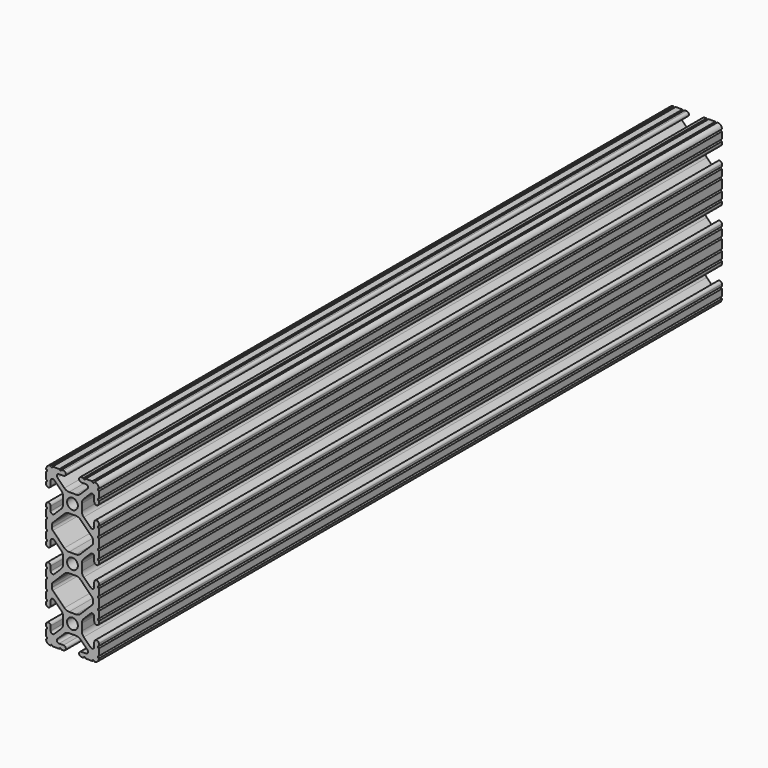
from build123d import *

# Parameters (mm, degrees)
F1_DEPTH = 375


# Not quite as in the source:
# - ends of sketch curves that miss each other by under 0.0002 mm in the source are joined


with BuildPart() as f1:
    # F0 (on Front) → F1 (new body)
    with BuildSketch(Plane.XZ):
        with BuildLine():
            ThreePointArc((-9.5504, 38.1), (-10.0584, 37.592), (-10.5664, 38.1))
            ThreePointArc((-10.5664, 38.1), (-12.0826749161, 37.4826749161), (-12.699997541, 35.9664000298))
            ThreePointArc((-12.699997541, 35.9664000298), (-12.192, 35.4584), (-12.7, 34.9504))
            Line((-12.7, 34.9504), (-12.7, 31.7246))
            ThreePointArc((-12.7, 31.7246), (-12.192, 31.2166), (-12.7, 30.7086))
            Line((-12.7, 30.7086), (-12.7, 29.7023028))
            ThreePointArc((-12.7, 29.7023028), (-11.5951, 28.5974028), (-10.4902, 29.7023028))
            Line((-10.4902, 29.7023028), (-10.4902, 31.8747902))
            ThreePointArc((-10.4902, 31.8747902), (-9.8630063673, 32.813451805), (-8.7557795103, 32.5932106897))
            Line((-8.7557795103, 32.5932106897), (-5.4384448, 29.2758622))
            ThreePointArc((-5.4384448, 29.2758622), (-4.7501824843, 28.2458268978), (-4.5085, 27.030807))
            Line((-4.5085, 27.030807), (-4.5085, 23.769193))
            ThreePointArc((-4.5085, 23.769193), (-4.7501824843, 22.5541731022), (-5.4384359697, 21.5241289697))
            Line((-5.4384359697, 21.5241289697), (-8.7557864, 18.2067962))
            ThreePointArc((-8.7557864, 18.2067962), (-9.8630063673, 17.986548195), (-10.4902, 18.9252098))
            Line((-10.4902, 18.9252098), (-10.4902, 21.0976972))
            ThreePointArc((-10.4902, 21.0976972), (-11.5951, 22.2025972), (-12.7, 21.0976972))
            Line((-12.7, 21.0976972), (-12.7, 20.0914))
            ThreePointArc((-12.7, 20.0914), (-12.192, 19.5834), (-12.7, 19.0754))
            Line((-12.7, 19.0754), (-12.7, 15.8496))
            ThreePointArc((-12.7, 15.8496), (-12.192, 15.3416), (-12.7, 14.8336))
            Line((-12.7, 14.8336), (-12.7, 10.5664))
            ThreePointArc((-12.7, 10.5664), (-12.192, 10.0584), (-12.7, 9.5504))
            Line((-12.7, 9.5504), (-12.7, 6.3246))
            ThreePointArc((-12.7, 6.3246), (-12.192, 5.8166), (-12.7, 5.3086))
            Line((-12.7, 5.3086), (-12.7, 4.3023028))
            ThreePointArc((-12.7, 4.3023028), (-11.5951, 3.1974028), (-10.4902, 4.3023028))
            Line((-10.4902, 4.3023028), (-10.4902, 6.4747902))
            ThreePointArc((-10.4902, 6.4747902), (-9.8630063673, 7.413451805), (-8.7557795103, 7.1932106897))
            Line((-8.7557795103, 7.1932106897), (-5.4384448, 3.8758622))
            ThreePointArc((-5.4384448, 3.8758622), (-4.7501824843, 2.8458268978), (-4.5085, 1.630807))
            Line((-4.5085, 1.630807), (-4.5085, -1.630807))
            ThreePointArc((-4.5085, -1.630807), (-4.7501824843, -2.8458268978), (-5.4384359697, -3.8758710303))
            Line((-5.4384359697, -3.8758710303), (-8.7557864, -7.1932038))
            ThreePointArc((-8.7557864, -7.1932038), (-9.8630063673, -7.413451805), (-10.4902, -6.4747902))
            Line((-10.4902, -6.4747902), (-10.4902, -4.3023028))
            ThreePointArc((-10.4902, -4.3023028), (-11.5951, -3.1974028), (-12.7, -4.3023028))
            Line((-12.7, -4.3023028), (-12.7, -5.3086))
            ThreePointArc((-12.7, -5.3086), (-12.192, -5.8166), (-12.7, -6.3246))
            Line((-12.7, -6.3246), (-12.7, -9.5504))
            ThreePointArc((-12.7, -9.5504), (-12.192, -10.0584), (-12.7, -10.5664))
            Line((-12.7, -10.5664), (-12.7, -14.8336))
            ThreePointArc((-12.7, -14.8336), (-12.192, -15.3416), (-12.7, -15.8496))
            Line((-12.7, -15.8496), (-12.7, -19.0754))
            ThreePointArc((-12.7, -19.0754), (-12.192, -19.5834), (-12.7, -20.0914))
            Line((-12.7, -20.0914), (-12.7, -21.0976972))
            ThreePointArc((-12.7, -21.0976972), (-11.5951, -22.2025972), (-10.4902, -21.0976972))
            Line((-10.4902, -21.0976972), (-10.4902, -18.9252098))
            ThreePointArc((-10.4902, -18.9252098), (-9.8630063673, -17.986548195), (-8.7557795103, -18.2067893103))
            Line((-8.7557795103, -18.2067893103), (-5.4384448, -21.5241378))
            ThreePointArc((-5.4384448, -21.5241378), (-4.7501824843, -22.5541731022), (-4.5085, -23.769193))
            Line((-4.5085, -23.769193), (-4.5085, -27.030807))
            ThreePointArc((-4.5085, -27.030807), (-4.7501824843, -28.2458268978), (-5.4384359697, -29.2758710303))
            Line((-5.4384359697, -29.2758710303), (-8.7557864, -32.5932038))
            ThreePointArc((-8.7557864, -32.5932038), (-9.8630063673, -32.813451805), (-10.4902, -31.8747902))
            Line((-10.4902, -31.8747902), (-10.4902, -29.7023028))
            ThreePointArc((-10.4902, -29.7023028), (-11.5951, -28.5974028), (-12.7, -29.7023028))
            Line((-12.7, -29.7023028), (-12.7, -30.7086))
            ThreePointArc((-12.7, -30.7086), (-12.192, -31.2166), (-12.7, -31.7246))
            Line((-12.7, -31.7246), (-12.7, -34.9504))
            ThreePointArc((-12.7, -34.9504), (-12.192, -35.4584), (-12.7, -35.9664))
            ThreePointArc((-12.7, -35.9664), (-12.0826749161, -37.4826749161), (-10.5664000298, -38.099997541))
            ThreePointArc((-10.5664000298, -38.099997541), (-10.0584, -37.592), (-9.5504, -38.1))
            Line((-9.5504, -38.1), (-6.3246, -38.1))
            ThreePointArc((-6.3246, -38.1), (-5.8166, -37.592), (-5.3086, -38.1))
            Line((-5.3086, -38.1), (-4.3023028, -38.1))
            ThreePointArc((-4.3023028, -38.1), (-3.1974028, -36.9951), (-4.3023028, -35.8902))
            Line((-4.3023028, -35.8902), (-6.4747902, -35.8902))
            ThreePointArc((-6.4747902, -35.8902), (-7.413451805, -35.2630063673), (-7.1932106897, -34.1557795103))
            Line((-7.1932106897, -34.1557795103), (-3.8758622, -30.8384448))
            ThreePointArc((-3.8758622, -30.8384448), (-2.8458268978, -30.1501824843), (-1.630807, -29.9085))
            Line((-1.630807, -29.9085), (1.630807, -29.9085))
            ThreePointArc((1.630807, -29.9085), (2.8458268978, -30.1501824843), (3.8758710303, -30.8384359697))
            Line((3.8758710303, -30.8384359697), (7.1932038, -34.1557864))
            ThreePointArc((7.1932038, -34.1557864), (7.413451805, -35.2630063673), (6.4747902, -35.8902))
            Line((6.4747902, -35.8902), (4.3023028, -35.8902))
            ThreePointArc((4.3023028, -35.8902), (3.1974028, -36.9951), (4.3023028, -38.1))
            Line((4.3023028, -38.1), (5.3086, -38.1))
            ThreePointArc((5.3086, -38.1), (5.8166, -37.592), (6.3246, -38.1))
            Line((6.3246, -38.1), (9.5504, -38.1))
            ThreePointArc((9.5504, -38.1), (10.0584, -37.592), (10.5664, -38.1))
            ThreePointArc((10.5664, -38.1), (12.0826749161, -37.4826749161), (12.699997541, -35.9664000298))
            ThreePointArc((12.699997541, -35.9664000298), (12.192, -35.4584), (12.7, -34.9504))
            Line((12.7, -34.9504), (12.7, -31.7246))
            ThreePointArc((12.7, -31.7246), (12.192, -31.2166), (12.7, -30.7086))
            Line((12.7, -30.7086), (12.7, -29.7023028))
            ThreePointArc((12.7, -29.7023028), (11.5951, -28.5974028), (10.4902, -29.7023028))
            Line((10.4902, -29.7023028), (10.4902, -31.8747902))
            ThreePointArc((10.4902, -31.8747902), (9.8630063673, -32.813451805), (8.7557795103, -32.5932106897))
            Line((8.7557795103, -32.5932106897), (5.4384448, -29.2758622))
            ThreePointArc((5.4384448, -29.2758622), (4.7501824843, -28.2458268978), (4.5085, -27.030807))
            Line((4.5085, -27.030807), (4.5085, -23.769193))
            ThreePointArc((4.5085, -23.769193), (4.7501824843, -22.5541731022), (5.4384359697, -21.5241289697))
            Line((5.4384359697, -21.5241289697), (8.7557864, -18.2067962))
            ThreePointArc((8.7557864, -18.2067962), (9.8630063673, -17.986548195), (10.4902, -18.9252098))
            Line((10.4902, -18.9252098), (10.4902, -21.0976972))
            ThreePointArc((10.4902, -21.0976972), (11.5951, -22.2025972), (12.7, -21.0976972))
            Line((12.7, -21.0976972), (12.7, -20.0914))
            ThreePointArc((12.7, -20.0914), (12.192, -19.5834), (12.7, -19.0754))
            Line((12.7, -19.0754), (12.7, -15.8496))
            ThreePointArc((12.7, -15.8496), (12.192, -15.3416), (12.7, -14.8336))
            Line((12.7, -14.8336), (12.7, -10.5664))
            ThreePointArc((12.7, -10.5664), (12.192, -10.0584), (12.7, -9.5504))
            Line((12.7, -9.5504), (12.7, -6.3246))
            ThreePointArc((12.7, -6.3246), (12.192, -5.8166), (12.7, -5.3086))
            Line((12.7, -5.3086), (12.7, -4.3023028))
            ThreePointArc((12.7, -4.3023028), (11.5951, -3.1974028), (10.4902, -4.3023028))
            Line((10.4902, -4.3023028), (10.4902, -6.4747902))
            ThreePointArc((10.4902, -6.4747902), (9.8630063673, -7.413451805), (8.7557795103, -7.1932106897))
            Line((8.7557795103, -7.1932106897), (5.4384448, -3.8758622))
            ThreePointArc((5.4384448, -3.8758622), (4.7501824843, -2.8458268978), (4.5085, -1.630807))
            Line((4.5085, -1.630807), (4.5085, 1.630807))
            ThreePointArc((4.5085, 1.630807), (4.7501824843, 2.8458268978), (5.4384359697, 3.8758710303))
            Line((5.4384359697, 3.8758710303), (8.7557864, 7.1932038))
            ThreePointArc((8.7557864, 7.1932038), (9.8630063673, 7.413451805), (10.4902, 6.4747902))
            Line((10.4902, 6.4747902), (10.4902, 4.3023028))
            ThreePointArc((10.4902, 4.3023028), (11.5951, 3.1974028), (12.7, 4.3023028))
            Line((12.7, 4.3023028), (12.7, 5.3086))
            ThreePointArc((12.7, 5.3086), (12.192, 5.8166), (12.7, 6.3246))
            Line((12.7, 6.3246), (12.7, 9.5504))
            ThreePointArc((12.7, 9.5504), (12.192, 10.0584), (12.7, 10.5664))
            Line((12.7, 10.5664), (12.7, 14.8336))
            ThreePointArc((12.7, 14.8336), (12.192, 15.3416), (12.7, 15.8496))
            Line((12.7, 15.8496), (12.7, 19.0754))
            ThreePointArc((12.7, 19.0754), (12.192, 19.5834), (12.7, 20.0914))
            Line((12.7, 20.0914), (12.7, 21.0976972))
            ThreePointArc((12.7, 21.0976972), (11.5951, 22.2025972), (10.4902, 21.0976972))
            Line((10.4902, 21.0976972), (10.4902, 18.9252098))
            ThreePointArc((10.4902, 18.9252098), (9.8630063673, 17.986548195), (8.7557795103, 18.2067893103))
            Line((8.7557795103, 18.2067893103), (5.4384448, 21.5241378))
            ThreePointArc((5.4384448, 21.5241378), (4.7501824843, 22.5541731022), (4.5085, 23.769193))
            Line((4.5085, 23.769193), (4.5085, 27.030807))
            ThreePointArc((4.5085, 27.030807), (4.7501824843, 28.2458268978), (5.4384359697, 29.2758710303))
            Line((5.4384359697, 29.2758710303), (8.7557864, 32.5932038))
            ThreePointArc((8.7557864, 32.5932038), (9.8630063673, 32.813451805), (10.4902, 31.8747902))
            Line((10.4902, 31.8747902), (10.4902, 29.7023028))
            ThreePointArc((10.4902, 29.7023028), (11.5951, 28.5974028), (12.7, 29.7023028))
            Line((12.7, 29.7023028), (12.7, 30.7086))
            ThreePointArc((12.7, 30.7086), (12.192, 31.2166), (12.7, 31.7246))
            Line((12.7, 31.7246), (12.7, 34.9504))
            ThreePointArc((12.7, 34.9504), (12.192, 35.4584), (12.7, 35.9664))
            ThreePointArc((12.7, 35.9664), (12.0826749161, 37.4826749161), (10.5664000298, 38.099997541))
            ThreePointArc((10.5664000298, 38.099997541), (10.0584, 37.592), (9.5504, 38.1))
            Line((9.5504, 38.1), (6.3246, 38.1))
            ThreePointArc((6.3246, 38.1), (5.8166, 37.592), (5.3086, 38.1))
            Line((5.3086, 38.1), (4.3023028, 38.1))
            ThreePointArc((4.3023028, 38.1), (3.1974028, 36.9951), (4.3023028, 35.8902))
            Line((4.3023028, 35.8902), (6.4747902, 35.8902))
            ThreePointArc((6.4747902, 35.8902), (7.413451805, 35.2630063673), (7.1932106897, 34.1557795103))
            Line((7.1932106897, 34.1557795103), (3.8758622, 30.8384448))
            ThreePointArc((3.8758622, 30.8384448), (2.8458268978, 30.1501824843), (1.630807, 29.9085))
            Line((1.630807, 29.9085), (-1.630807, 29.9085))
            ThreePointArc((-1.630807, 29.9085), (-2.8458268978, 30.1501824843), (-3.8758710303, 30.8384359697))
            Line((-3.8758710303, 30.8384359697), (-7.1932038, 34.1557864))
            ThreePointArc((-7.1932038, 34.1557864), (-7.413451805, 35.2630063673), (-6.4747902, 35.8902))
            Line((-6.4747902, 35.8902), (-4.3023028, 35.8902))
            ThreePointArc((-4.3023028, 35.8902), (-3.1974028, 36.9951), (-4.3023028, 38.1))
            Line((-4.3023028, 38.1), (-5.3086, 38.1))
            ThreePointArc((-5.3086, 38.1), (-5.8166, 37.592), (-6.3246, 38.1))
            Line((-6.3246, 38.1), (-9.5504, 38.1))
        make_face()
        with BuildLine():
            ThreePointArc((-2.6035, -25.4), (0, -22.7965), (2.6035, -25.4))
            ThreePointArc((2.6035, -25.4), (0, -28.0035), (-2.6035, -25.4))
        make_face(mode=Mode.SUBTRACT)
        with BuildLine():
            Line((-9.4701614, -11.0327186), (-3.8758622, -5.4384448))
            ThreePointArc((-3.8758622, -5.4384448), (-2.8458268978, -4.7501824843), (-1.630807, -4.5085))
            Line((-1.630807, -4.5085), (1.630807, -4.5085))
            ThreePointArc((1.630807, -4.5085), (2.8458268978, -4.7501824843), (3.8758710303, -5.4384359697))
            Line((3.8758710303, -5.4384359697), (9.4701614, -11.0327186))
            ThreePointArc((9.4701614, -11.0327186), (9.8115254878, -11.5436301307), (9.9314, -12.14628))
            Line((9.9314, -12.14628), (9.9314, -13.25372))
            ThreePointArc((9.9314, -13.25372), (9.8115254878, -13.8563698693), (9.470151759, -14.367271759))
            Line((9.470151759, -14.367271759), (3.8758622, -19.9615552))
            ThreePointArc((3.8758622, -19.9615552), (2.8458268978, -20.6498175157), (1.630807, -20.8915))
            Line((1.630807, -20.8915), (-1.630807, -20.8915))
            ThreePointArc((-1.630807, -20.8915), (-2.8458268978, -20.6498175157), (-3.8758710303, -19.9615640303))
            Line((-3.8758710303, -19.9615640303), (-9.4701614, -14.3672814))
            ThreePointArc((-9.4701614, -14.3672814), (-9.8115254878, -13.8563698693), (-9.9314, -13.25372))
            Line((-9.9314, -13.25372), (-9.9314, -12.14628))
            ThreePointArc((-9.9314, -12.14628), (-9.8115254878, -11.5436301307), (-9.4701614, -11.0327186))
        make_face(mode=Mode.SUBTRACT)
        with BuildLine():
            ThreePointArc((-2.6035, 0), (0, 2.6035), (2.6035, 0))
            ThreePointArc((2.6035, 0), (0, -2.6035), (-2.6035, 0))
        make_face(mode=Mode.SUBTRACT)
        with BuildLine():
            Line((-9.4701614, 14.3672814), (-3.8758622, 19.9615552))
            ThreePointArc((-3.8758622, 19.9615552), (-2.8458268978, 20.6498175157), (-1.630807, 20.8915))
            Line((-1.630807, 20.8915), (1.630807, 20.8915))
            ThreePointArc((1.630807, 20.8915), (2.8458268978, 20.6498175157), (3.8758710303, 19.9615640303))
            Line((3.8758710303, 19.9615640303), (9.4701614, 14.3672814))
            ThreePointArc((9.4701614, 14.3672814), (9.8115254878, 13.8563698693), (9.9314, 13.25372))
            Line((9.9314, 13.25372), (9.9314, 12.14628))
            ThreePointArc((9.9314, 12.14628), (9.8115254878, 11.5436301307), (9.470151759, 11.032728241))
            Line((9.470151759, 11.032728241), (3.8758622, 5.4384448))
            ThreePointArc((3.8758622, 5.4384448), (2.8458268978, 4.7501824843), (1.630807, 4.5085))
            Line((1.630807, 4.5085), (-1.630807, 4.5085))
            ThreePointArc((-1.630807, 4.5085), (-2.8458268978, 4.7501824843), (-3.8758710303, 5.4384359697))
            Line((-3.8758710303, 5.4384359697), (-9.4701614, 11.0327186))
            ThreePointArc((-9.4701614, 11.0327186), (-9.8115254878, 11.5436301307), (-9.9314, 12.14628))
            Line((-9.9314, 12.14628), (-9.9314, 13.25372))
            ThreePointArc((-9.9314, 13.25372), (-9.8115254878, 13.8563698693), (-9.4701614, 14.3672814))
        make_face(mode=Mode.SUBTRACT)
        with BuildLine():
            ThreePointArc((-2.6035, 25.4), (0, 28.0035), (2.6035, 25.4))
            ThreePointArc((2.6035, 25.4), (0, 22.7965), (-2.6035, 25.4))
        make_face(mode=Mode.SUBTRACT)
    extrude(amount=F1_DEPTH)


solid = f1.part
